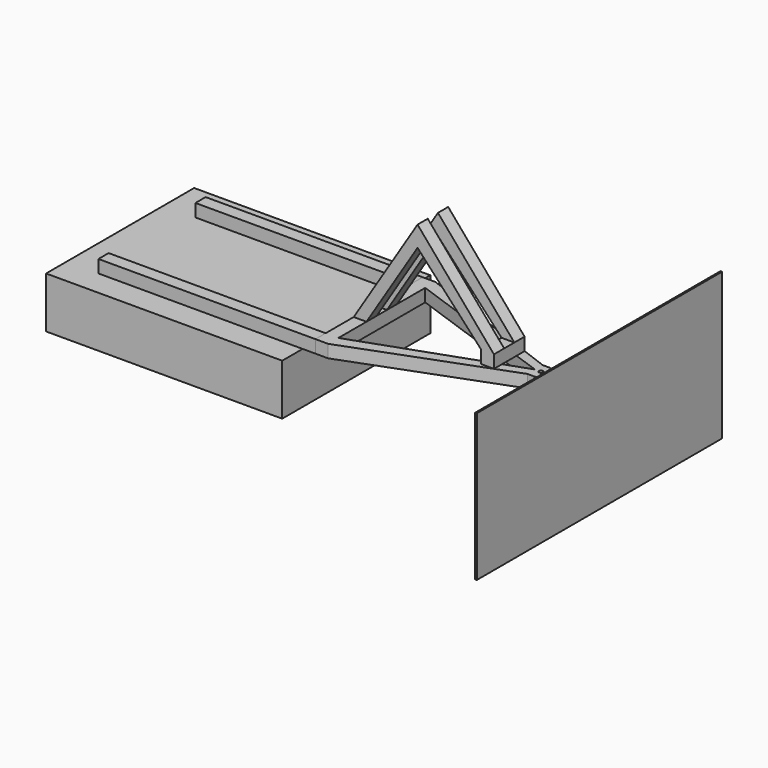
from build123d import *

# Parameters (mm, degrees)
F1_W      = 406.4
F1_H      = 25.4
F1_W_2    = 25.4
F2_DEPTH  = 25.4
F3_W      = 241.3
F3_H      = 25.4
F3_W_2    = 25.4
F4_DEPTH  = 25.4
F0_W      = 469.9
F0_H      = 368.3
F5_DEPTH  = 101.6
F6_R      = 3.96875
F7_DEPTH  = 25.4
F8_W      = 25.4
F8_H      = 457.2
F8_R      = 3.96875
F9_DEPTH  = 25.4
F10_W     = 25.4
F10_H     = 101.6
F10_R     = 3.96875
F11_DEPTH = 25.4
F12_W     = 609.6
F12_H     = 292.1
F12_W_2   = 457.2
F12_H_2   = 25.4
F13_DEPTH = 3.175
F14_R     = 12.7
F16_DEPTH = 25.4
F18_DEPTH = 25.4
F20_DEPTH = 25.4


# Not quite as in the source:
# - a feature names something its author has since deleted; it is built from what else it names


with BuildPart() as f2:
    # F1 (on face) → F2 (new body)
    with BuildSketch(Plane.XY):
        with Locations((31.75, -120.65)):
            Rectangle(F1_W, F1_H)
        with Locations((247.65, -120.65)):
            Rectangle(F1_W_2, F1_H)
    extrude(amount=F2_DEPTH)


with BuildPart() as f2b:
    # F1 (on face) → F2, piece 2 (new body)
    with BuildSketch(Plane.XY):
        with Locations((31.75, 120.65)):
            Rectangle(F1_W, F1_H)
        with Locations((247.65, 120.65)):
            Rectangle(F1_W_2, F1_H)
    extrude(amount=F2_DEPTH)


with BuildPart() as f4:
    # F3 (on face) → F4 (new body)
    with BuildSketch(Plane.YZ.offset(260.35)):
        with Locations((12.7, 12.7)):
            Rectangle(F3_W, F3_H)
        with Locations((-120.65, 12.7)):
            Rectangle(F3_W_2, F3_H)
    extrude(amount=F4_DEPTH)

    # F6 (on face) → F7 (join)
    with BuildSketch(Plane.XY):
        Polygon((285.75, -107.95), (285.75, -133.35), (590.55, -19.05), (590.55, 0), align=None)
        Polygon((590.55, 19.05), (285.75, 133.35), (285.75, 107.95), (590.55, 0), align=None)
        Polygon((615.95, 19.05), (590.55, 19.05), (590.55, 0), (590.55, -19.05), (615.95, -19.05), align=None)
        with Locations((602.4379256336, 0)):
            Circle(F6_R, mode=Mode.SUBTRACT)
    extrude(amount=F7_DEPTH)

    # F14
    f14_edges = [f4.edges().sort_by_distance(p)[0] for p in [
        (615.95, 19.05, 12.7),
        (615.95, -19.05, 12.7),
    ]]
    fillet(f14_edges, radius=F14_R)

    # F15 (on face) → F16 (join)
    with BuildSketch(Plane.XY.offset(25.4)):
        Polygon((539.3700387001, -18.1262362937), (513.9700387001, -27.122069627), (513.9700387001, -38.1), (539.3700387001, -38.1), align=None)
        Polygon((539.3700387001, 18.1262362937), (513.9700387001, 27.122069627), (513.9700387001, -27.122069627), (539.3700387001, -18.1262362937), align=None)
        Polygon((539.3700387001, 38.1), (513.9700387001, 38.1), (513.9700387001, 27.122069627), (539.3700387001, 18.1262362937), align=None)
    extrude(amount=F16_DEPTH)

    # F17 (on face) → F18 (join)
    with BuildSketch(Plane.XZ.offset(38.1)):
        Polygon((260.35, 25.4), (285.75, 25.4), (387.35, 187.96), (513.9700387001, 50.8), (539.3700387001, 50.8), (387.35, 228.6), align=None)
    extrude(amount=-F18_DEPTH)

    # F19 (on face) → F20 (join)
    with BuildSketch(Plane(origin=(0, 38.1, 0), x_dir=(-1, 0, 0), z_dir=(0, 1, 0))):
        Polygon((-539.3700387001, 50.8), (-513.9700387001, 50.8), (-387.35, 187.96), (-285.75, 25.4), (-260.35, 25.4), (-387.35, 228.6), align=None)
    extrude(amount=-F20_DEPTH)


with BuildPart() as f5:
    # F0 (on Top) → F5 (new body)
    with BuildSketch(Plane.XY):
        Rectangle(F0_W, F0_H)
    extrude(amount=-F5_DEPTH)


with BuildPart() as f9:
    # F8 (on face) → F9 (new body)
    with BuildSketch(Plane.XY.offset(25.4)):
        with Locations((702.8098106384, 0)):
            Rectangle(F8_W, F8_H)
        with Locations((702.8098106384, 0)):
            Circle(F8_R, mode=Mode.SUBTRACT)
    extrude(amount=F9_DEPTH)


with BuildPart() as f11:
    # F10 (on face) → F11 (new body)
    with BuildSketch(Plane(origin=(0, 0, 0), x_dir=(1, 0, 0), z_dir=(0, 0, -1))):
        with Locations((702.8098106384, 0)):
            Rectangle(F10_W, F10_H)
        with Locations((702.8098106384, 0)):
            Circle(F10_R, mode=Mode.SUBTRACT)
    extrude(amount=F11_DEPTH)

    # F12 (on face) → F13 (join)
    with BuildSketch(Plane.YZ.offset(715.5098106384)):
        with Locations((0, -31.75)):
            Rectangle(F12_W, F12_H)
        with Locations((0, 38.1)):
            Rectangle(F12_W_2, F12_H_2, mode=Mode.SUBTRACT)
        with Locations((0, 38.1)):
            Rectangle(F12_W_2, F12_H_2)
    extrude(amount=F13_DEPTH)


solid = Compound([f2.part, f2b.part, f4.part, f5.part, f9.part, f11.part])
